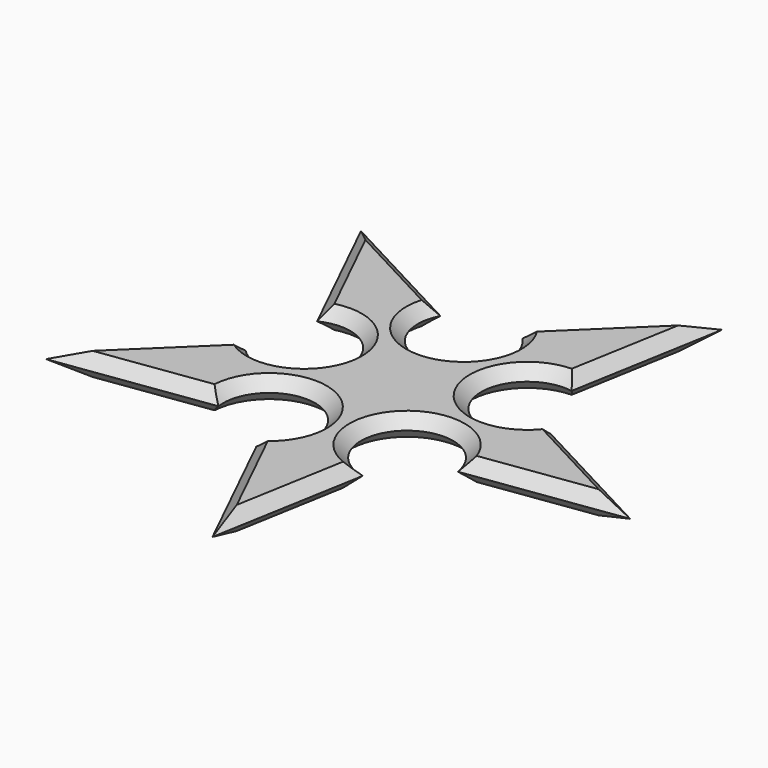
from build123d import *

# Parameters (mm, degrees)
F1_DEPTH = 4.7625
F2_R     = 9.525
F3_DEPTH = 4.7635
F4_SIZE  = 2.38124


# Not quite as in the source:
# - a fillet or chamfer is up to 0.001 mm smaller than in the source, because OpenCascade refuses the exact size
# - a feature of the source that left no trace in its solid (it failed there, or was rolled back) is left out


with BuildPart() as f1:
    # F0 (on Top) → F1 (new body)
    with BuildSketch(Plane.XY):
        Polygon((-3.074264621, 21.805118867), (-40.0660246394, 41.4531760826), (-21.6879004002, 3.8143528936), (-51.8053957451, -25.295317935), (-10.3295949709, -19.4477191337), (8.0485292683, -57.0865423226), (15.3038596181, -15.8337043219), (56.7796603923, -9.9861055206), (19.787900374, 9.6619516949), (27.0432307238, 50.9147896956), align=None)
    extrude(amount=F1_DEPTH)

    # F2 (on Top) → F3 (cut, through all)
    with BuildSketch(Plane.XY):
        with Locations((15.3038596181, -15.8337043219)):
            Circle(F2_R)
        with Locations((-10.3295949709, -19.4477191337)):
            Circle(F2_R)
        with Locations((-21.6879004002, 3.8143528936)):
            Circle(F2_R)
        with Locations((-3.074264621, 21.805118867)):
            Circle(F2_R)
        with Locations((19.787900374, 9.6619516949)):
            Circle(F2_R)
    extrude(amount=F3_DEPTH, mode=Mode.SUBTRACT)

    # F4 (size 2.38125 in the source; OpenCascade refuses exactly that, so slightly less here)
    f4_edges = [f1.edges().sort_by_distance(p)[0] for p in [
        (24.240507, 34.97888, 4.7625),
        (15.408887, 39.669767, 4.7625),
        (-1.744503, 12.373398, 4.7625),
        (-25.776163, 33.863161, 4.7625),
        (-32.966583, 26.913355, 4.7625),
        (-12.306882, 2.164469, 4.7625),
        (-40.171052, -14.050296, 4.7625),
        (-35.783356, -23.036399, 4.7625),
        (-5.861568, -11.035682, 4.7625),
        (0.949087, -42.546721, 4.7625),
        (10.851253, -41.150633, 4.7625),
        (8.684234, -8.984896, 4.7625),
        (40.75762, -12.245024, 4.7625),
        (42.489799, -2.39609, 4.7625),
        (11.22872, 5.482711, 4.7625),
        (24.240507, 34.97888, 0),
        (15.408887, 39.669767, 0),
        (-1.744503, 12.373398, 0),
        (-25.776163, 33.863161, 0),
        (-32.966583, 26.913355, 0),
        (-12.306882, 2.164469, 0),
        (-40.171052, -14.050296, 0),
        (-35.783356, -23.036399, 0),
        (-5.861568, -11.035682, 0),
        (0.949087, -42.546721, 0),
        (10.851253, -41.150633, 0),
        (8.684234, -8.984896, 0),
        (40.75762, -12.245024, 0),
        (42.489799, -2.39609, 0),
        (11.22872, 5.482711, 0),
    ]]
    chamfer(f4_edges, length=F4_SIZE)


solid = f1.part
